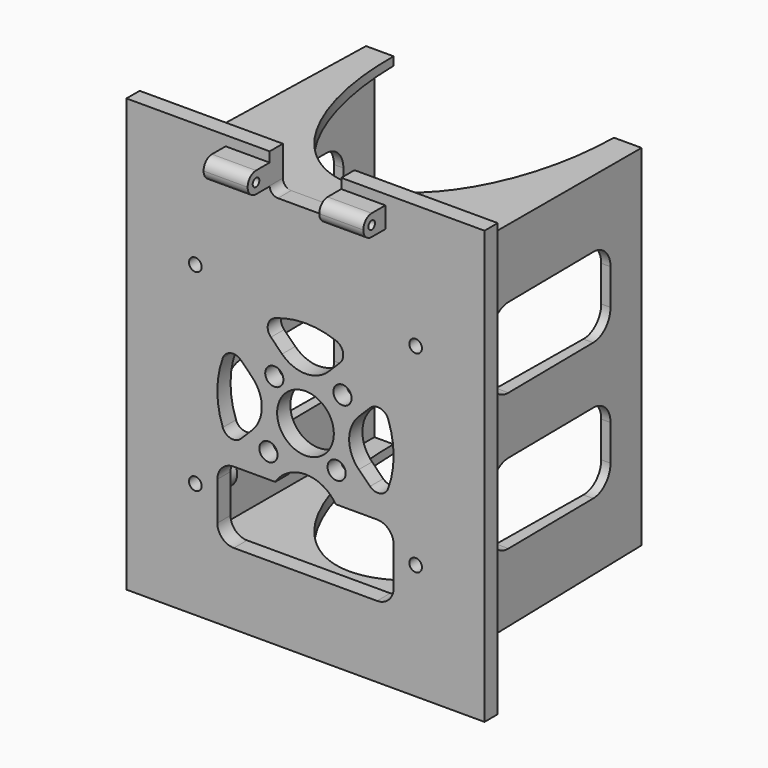
from build123d import *

# Parameters (mm, degrees)
F0_R           = 1.15
F0_R_2         = 1.65
F0_R_3         = 5.15
F1_DEPTH       = 3
F2_W           = 46
F2_H           = 59.5
F3_DEPTH       = 42
F3_TAPER       = 0.67
F2_R           = 2.8
F2_R_2         = 1.15
F4_DEPTH       = 3
F6_DEPTH       = 71.5
F8_DEPTH       = 26.4140474431
F8_DEPTH_BACK  = 26.4140474431
F10_DEPTH      = 5
F11_R          = 1.89999
F12_R          = 0.75
F13_DEPTH      = 25
F13_DEPTH_BACK = 25


# Not quite as in the source:
# - a fillet or chamfer is up to 0.001 mm smaller than in the source, because OpenCascade refuses the exact size


with BuildPart() as f1:
    # F0 (on Front) → F1 (new body)
    with BuildSketch(Plane.XZ):
        with BuildLine():
            Line((-32.5, 78.5), (-32.5, 0))
            Line((-32.5, 0), (32.5, 0))
            Line((32.5, 0), (32.5, 78.5))
            Line((32.5, 78.5), (6.5, 78.5))
            Line((6.5, 78.5), (6.5, 73))
            ThreePointArc((6.5, 73), (6.0606601718, 71.9393398282), (5, 71.5))
            Line((5, 71.5), (0, 71.5))
            Line((0, 71.5), (-5, 71.5))
            ThreePointArc((-5, 71.5), (-6.0606601718, 71.9393398282), (-6.5, 73))
            Line((-6.5, 73), (-6.5, 78.5))
            Line((-6.5, 78.5), (-32.5, 78.5))
        make_face()
        with Locations((-20, 21)):
            Circle(F0_R, mode=Mode.SUBTRACT)
        with BuildLine():
            ThreePointArc((-11.7161784284, 30.8785437868), (-13.558147189, 30.3390364145), (-15.0061622751, 31.5988655419))
            ThreePointArc((-15.0061622751, 31.5988655419), (-16, 37.15), (-15.0061622751, 42.7011344581))
            ThreePointArc((-15.0061622751, 42.7011344581), (-13.558147189, 43.9609635855), (-11.7161784284, 43.4214562132))
            Line((-11.7161784284, 43.4214562132), (-9.6873629023, 41.3926406871))
            ThreePointArc((-9.6873629023, 41.3926406871), (-7.9300035894, 37.15), (-9.6873629023, 32.9073593129))
            Line((-9.6873629023, 32.9073593129), (-11.7161784284, 30.8785437868))
        make_face(mode=Mode.SUBTRACT)
        with Locations((-6.7175144213, 30.4324855787)):
            Circle(F0_R_2, mode=Mode.SUBTRACT)
        with BuildLine():
            ThreePointArc((-16, 23), (-15.1213203436, 25.1213203436), (-13, 26))
            Line((-13, 26), (-5.5, 26))
            ThreePointArc((-5.5, 26), (0, 29), (5.5, 26))
            Line((5.5, 26), (13, 26))
            ThreePointArc((13, 26), (15.1213203436, 25.1213203436), (16, 23))
            Line((16, 23), (16, 16))
            ThreePointArc((16, 16), (15.1213203436, 13.8786796564), (13, 13))
            Line((13, 13), (-13, 13))
            ThreePointArc((-13, 13), (-15.1213203436, 13.8786796564), (-16, 16))
            Line((-16, 16), (-16, 23))
        make_face(mode=Mode.SUBTRACT)
        with Locations((5.6568542495, 31.4931457505)):
            Circle(F0_R_2, mode=Mode.SUBTRACT)
        with Locations((0, 37.15)):
            Circle(F0_R_3, mode=Mode.SUBTRACT)
        with BuildLine():
            ThreePointArc((11.7161784284, 43.4214562132), (13.558147189, 43.9609635855), (15.0061622751, 42.7011344581))
            ThreePointArc((15.0061622751, 42.7011344581), (16, 37.15), (15.0061622751, 31.5988655419))
            ThreePointArc((15.0061622751, 31.5988655419), (13.558147189, 30.3390364145), (11.7161784284, 30.8785437868))
            Line((11.7161784284, 30.8785437868), (9.6873629023, 32.9073593129))
            ThreePointArc((9.6873629023, 32.9073593129), (7.9300035894, 37.15), (9.6873629023, 41.3926406871))
            Line((9.6873629023, 41.3926406871), (11.7161784284, 43.4214562132))
        make_face(mode=Mode.SUBTRACT)
        with Locations((20, 21)):
            Circle(F0_R, mode=Mode.SUBTRACT)
        with Locations((-20, 56)):
            Circle(F0_R, mode=Mode.SUBTRACT)
        with Locations((-5.6568542495, 42.8068542495)):
            Circle(F0_R_2, mode=Mode.SUBTRACT)
        with Locations((6.7175144213, 43.8675144213)):
            Circle(F0_R_2, mode=Mode.SUBTRACT)
        with BuildLine():
            ThreePointArc((4.2426406871, 46.8373629023), (0, 45.0800035894), (-4.2426406871, 46.8373629023))
            Line((-4.2426406871, 46.8373629023), (-6.2714562132, 48.8661784284))
            ThreePointArc((-6.2714562132, 48.8661784284), (-6.8109635855, 50.708147189), (-5.5511344581, 52.1561622751))
            ThreePointArc((-5.5511344581, 52.1561622751), (0, 53.15), (5.5511344581, 52.1561622751))
            ThreePointArc((5.5511344581, 52.1561622751), (6.8109635855, 50.708147189), (6.2714562132, 48.8661784284))
            Line((6.2714562132, 48.8661784284), (4.2426406871, 46.8373629023))
        make_face(mode=Mode.SUBTRACT)
        with Locations((20, 56)):
            Circle(F0_R, mode=Mode.SUBTRACT)
    extrude(amount=F1_DEPTH)

    # F2 (on face) → F3 (join)
    with BuildSketch(Plane(origin=(0, 0, 0), x_dir=(-1, 0, 0), z_dir=(0, 1, 0))):
        Polygon((-5, 71.5), (-25.5, 71.5), (-25.5, 7), (25.5, 7), (25.5, 71.5), (5, 71.5), align=None)
        with Locations((0, 39.25)):
            Rectangle(F2_W, F2_H, mode=Mode.SUBTRACT)
    extrude(amount=F3_DEPTH, taper=F3_TAPER)

    # F2 (on face) → F4 (join)
    with BuildSketch(Plane(origin=(0, 0, 0), x_dir=(-1, 0, 0), z_dir=(0, 1, 0))):
        with Locations((-20, 56)):
            Circle(F2_R)
        with Locations((-20, 56)):
            Circle(F2_R_2, mode=Mode.SUBTRACT)
        with Locations((20, 56)):
            Circle(F2_R)
        with Locations((20, 56)):
            Circle(F2_R_2, mode=Mode.SUBTRACT)
        with Locations((20, 21)):
            Circle(F2_R)
        with Locations((20, 21)):
            Circle(F2_R_2, mode=Mode.SUBTRACT)
        with Locations((-20, 21)):
            Circle(F2_R)
        with Locations((-20, 21)):
            Circle(F2_R_2, mode=Mode.SUBTRACT)
    extrude(amount=F4_DEPTH)

    # F5 (on Top) → F6 (cut, through all)
    with BuildSketch(Plane.XY):
        with BuildLine():
            add(Edge.make_bspline(
                [(20, 42), (20, 102.6217782649), (-10, 72.3108891325), (-40, 42), (-10, 11.6891108675), (20, -18.6217782649), (20, 42)],
                knots=[4.7123889804, 4.7123889804, 4.7123889804, 6.8067840828, 6.8067840828, 8.9011791852, 8.9011791852, 10.9955742876, 10.9955742876, 10.9955742876], degree=2, weights=[1, 0.5, 1, 0.5, 1, 0.5, 1]))
        make_face()
    extrude(amount=F6_DEPTH, mode=Mode.SUBTRACT)

    # F7 (on Right) → F8 (cut, two sides)
    with BuildSketch(Plane.YZ) as f8_sk:
        with BuildLine():
            ThreePointArc((34.85, 54.95), (33.6784271247, 57.7784271247), (30.85, 58.95))
            Line((30.85, 58.95), (11.35, 58.95))
            ThreePointArc((11.35, 58.95), (8.5215728753, 57.7784271247), (7.35, 54.95))
            Line((7.35, 54.95), (7.35, 48.45))
            ThreePointArc((7.35, 48.45), (8.5215728753, 45.6215728753), (11.35, 44.45))
            Line((11.35, 44.45), (30.85, 44.45))
            ThreePointArc((30.85, 44.45), (33.6784271247, 45.6215728753), (34.85, 48.45))
            Line((34.85, 48.45), (34.85, 54.95))
        make_face()
        with BuildLine():
            ThreePointArc((11.35, 34.05), (8.5215728753, 32.8784271247), (7.35, 30.05))
            Line((7.35, 30.05), (7.35, 23.55))
            ThreePointArc((7.35, 23.55), (8.5215728753, 20.7215728753), (11.35, 19.55))
            Line((11.35, 19.55), (30.85, 19.55))
            ThreePointArc((30.85, 19.55), (33.6784271247, 20.7215728753), (34.85, 23.55))
            Line((34.85, 23.55), (34.85, 30.05))
            ThreePointArc((34.85, 30.05), (33.6784271247, 32.8784271247), (30.85, 34.05))
            Line((30.85, 34.05), (11.35, 34.05))
        make_face()
    extrude(amount=-F8_DEPTH, mode=Mode.SUBTRACT)
    extrude(f8_sk.sketch, amount=F8_DEPTH_BACK, mode=Mode.SUBTRACT)

    # F9 (on face) → F10 (join)
    with BuildSketch(Plane.XZ.offset(3)):
        Polygon((-6.5, 76.7), (-14.5, 76.7), (-14.5, 72.9), (-6.5, 72.9), (-6.5, 73), align=None)
        Polygon((6.5, 76.7), (6.5, 73), (6.5, 72.9), (14.5, 72.9), (14.5, 76.7), align=None)
    extrude(amount=F10_DEPTH)

    # F11 (radius 1.9 in the source; OpenCascade refuses exactly that, so slightly less here)
    f11_edges = [f1.edges().sort_by_distance(p)[0] for p in [
        (-10.5, -8, 72.9),
        (-10.5, -8, 76.7),
        (10.5, -8, 76.7),
        (10.5, -8, 72.9),
    ]]
    fillet(f11_edges, radius=F11_R)

    # F12 (on face) → F13 (cut, two sides)
    with BuildSketch(Plane.YZ.offset(-6.5)) as f13_sk:
        with Locations((-6.1, 74.8)):
            Circle(F12_R)
    extrude(amount=-F13_DEPTH, mode=Mode.SUBTRACT)
    extrude(f13_sk.sketch, amount=F13_DEPTH_BACK, mode=Mode.SUBTRACT)


solid = f1.part
